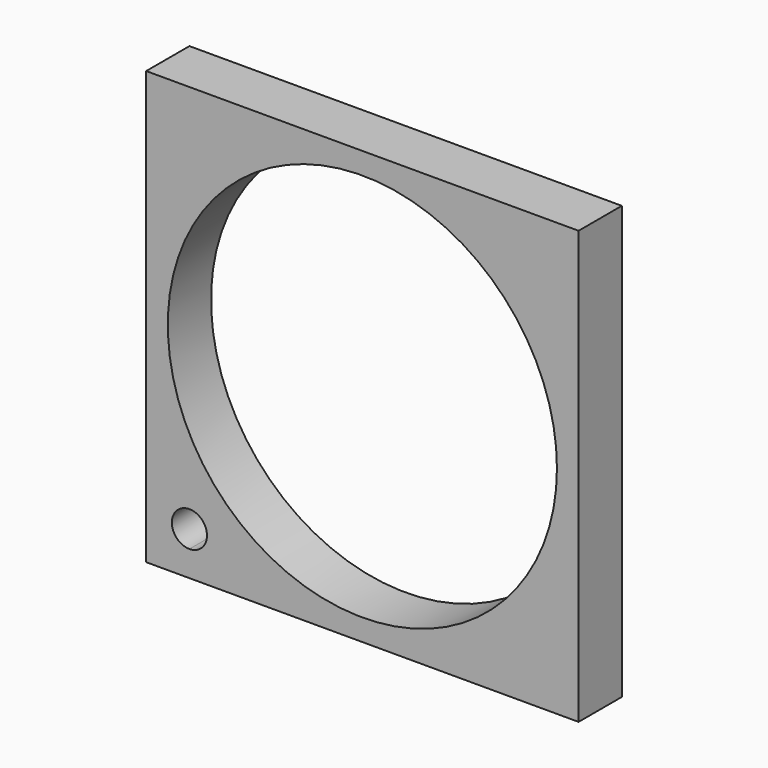
from build123d import *

# Parameters (mm, degrees)
F0_W     = 63.5
F0_H     = 63.5
F0_R     = 28.575
F1_DEPTH = 7.9375
F3_DEPTH = 25.4


# Not quite as in the source:
# - a length typed as a fraction of an inch, garbled in the dataset ("3 / 203.2 mm" for 3/8 in), is restored


with BuildPart() as f1:
    # F0 (on Front) → F1 (new body)
    with BuildSketch(Plane.XZ):
        Rectangle(F0_W, F0_H)
        Circle(F0_R, mode=Mode.SUBTRACT)
    extrude(amount=F1_DEPTH)

    # F2 (on face) → F3 (cut)
    with BuildSketch(Plane.XZ.offset(7.9375)):
        with BuildLine():
            ThreePointArc((-22.8203125, -25.4), (-27.2241145246, -23.5758854754), (-25.4, -27.9796875))
            ThreePointArc((-25.4, -27.9796875), (-23.5758854754, -27.2241145246), (-22.8203125, -25.4))
        make_face()
    extrude(amount=-F3_DEPTH, mode=Mode.SUBTRACT)


solid = f1.part
